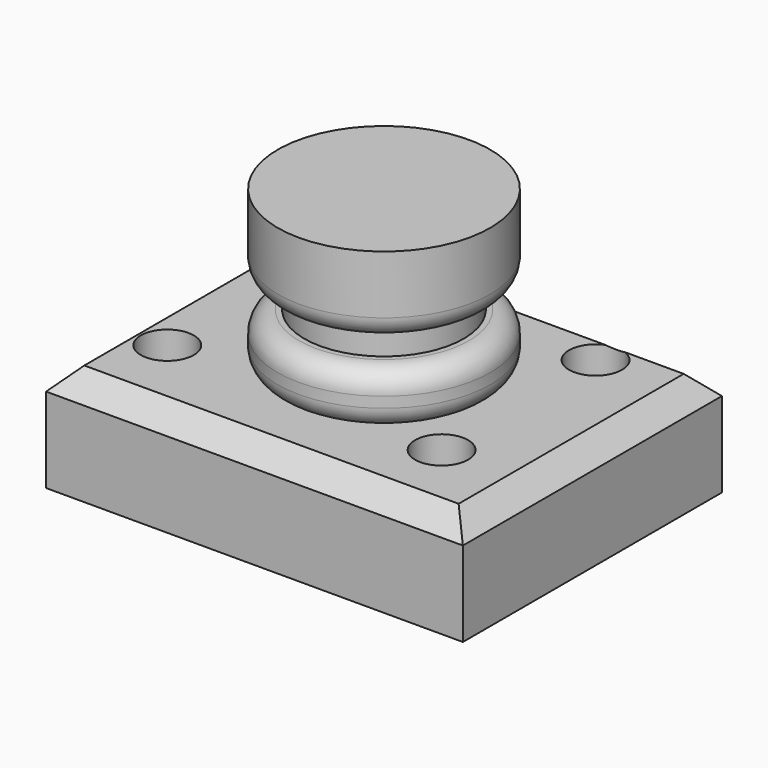
from build123d import *

# Parameters (mm, degrees)
F0_W        = 99.7109562159
F0_H        = 77.463619411
F0_R        = 6.35
F1_DEPTH    = 25.4
F2_W        = 25.4
F2_H        = 38.1
F4_W        = 18.3200901883
F4_H        = 6.35
F6_T1_DEPTH = 103.5919185687
F6_T3_DEPTH = 125.8392553736
F7_R        = 5.08
F8_R        = 5.08


# Not quite as in the source:
# - a fillet or chamfer that OpenCascade refuses, or shapes differently, is made with other operations: its cross-section is extruded or revolved along the edge and cut away or added


with BuildPart() as f1:
    # F0 (on Top) → F1 (new body)
    with BuildSketch(Plane.XY):
        Rectangle(F0_W, F0_H)
        with Locations((-37.7936698496, -17.5566338003)):
            Circle(F0_R, mode=Mode.SUBTRACT)
        with Locations((28.6803040653, -18.6287946999)):
            Circle(F0_R, mode=Mode.SUBTRACT)
        with Locations((-38.0617082119, 27.4741202593)):
            Circle(F0_R, mode=Mode.SUBTRACT)
        with Locations((28.4122619778, 27.7421604842)):
            Circle(F0_R, mode=Mode.SUBTRACT)
    extrude(amount=F1_DEPTH)

    # F6: chamfer of 5.08 on 4 edges, made by hand

    # F6_s2 → F6_t1 (cut)
    with BuildSketch(Plane.XZ.offset(-51.7959592844)):
        Polygon((49.8554781079, 20.32), (44.7754781079, 25.4), (49.8554781079, 25.4), align=None)
        Polygon((-49.8554781079, 20.32), (-44.7754781079, 25.4), (-49.8554781079, 25.4), align=None)
    extrude(amount=F6_T1_DEPTH, mode=Mode.SUBTRACT)

    # F6_s4 → F6_t3 (cut)
    with BuildSketch(Plane.YZ.offset(-62.9196276868)):
        Polygon((38.7318097055, 20.32), (33.6518097055, 25.4), (38.7318097055, 25.4), align=None)
        Polygon((-38.7318097055, 20.32), (-33.6518097055, 25.4), (-38.7318097055, 25.4), align=None)
    extrude(amount=F6_T3_DEPTH, mode=Mode.SUBTRACT)


with BuildPart() as f3:
    # F2 (on Right) → F3 (revolve)
    with BuildSketch(Plane.YZ):
        with Locations((-12.7, 44.45)):
            Rectangle(F2_W, F2_H)
    revolve(axis=Axis((0, 0, 44.45), (0, 0, -1)))

    # F4 (on Right) → F5 (revolve, cut)
    with BuildSketch(Plane.YZ):
        with Locations((-28.2100450942, 41.275)):
            Rectangle(F4_W, F4_H)
    revolve(axis=Axis((0, 0, 63.5), (0, 0, -1)), mode=Mode.SUBTRACT)

    # F7
    f7_edges = [f3.edges().sort_by_distance(p)[0] for p in [
        (0, 25.4, 38.1),
        (0, 25.4, 44.45),
    ]]
    fillet(f7_edges, radius=F7_R)

    # F8
    f8_edges = [f3.edges().sort_by_distance(p)[0] for p in [
        (0, 25.4, 25.4),
    ]]
    fillet(f8_edges, radius=F8_R)


solid = Compound([f1.part, f3.part])
